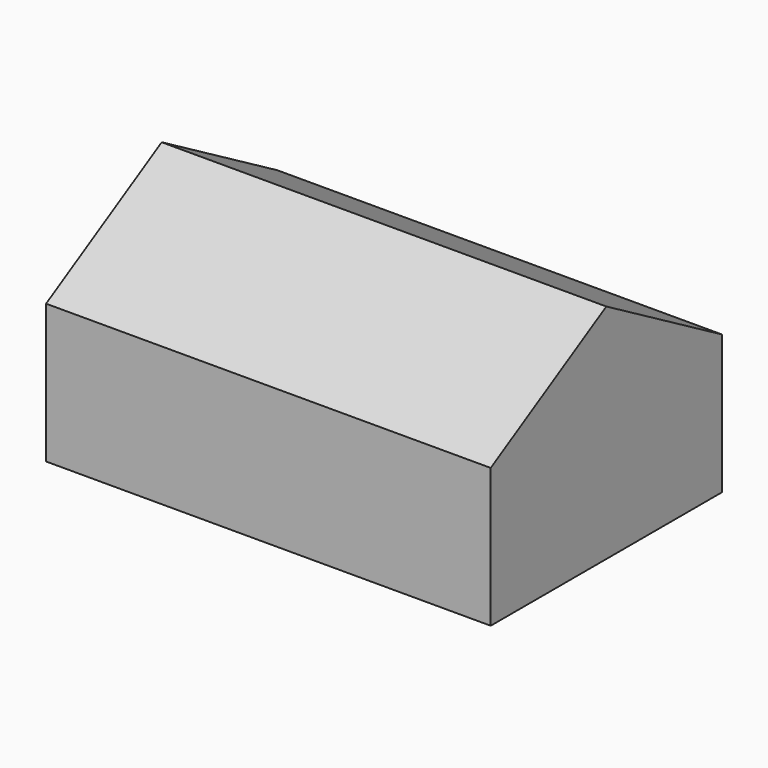
from build123d import *

# Parameters (mm, degrees)
F0_W     = 1250
F0_H     = 900
F0_W_2   = 900
F0_H_2   = 2055
F1_DEPTH = 8000


# Not quite as in the source:
# - the program builds the solid bodies; features that only make, move or delete a surface that nothing else refers to are left out


with BuildPart() as f1:
    # F0 (on Right) → F1 (new body)
    with BuildSketch(Plane.YZ):
        Polygon((-340, -1250), (2600, -1250), (2600, 1250), (0, 2750), (-2600, 1250), (-2600, -1250), (-1240, -1250), (-1240, 805), (-340, 805), align=None)
        with Locations((1175, 355)):
            Rectangle(F0_W, F0_H, mode=Mode.SUBTRACT)
        with Locations((-790, -222.5)):
            Rectangle(F0_W_2, F0_H_2)
        with Locations((1175, 355)):
            Rectangle(F0_W, F0_H)
    extrude(amount=F1_DEPTH)


solid = f1.part
